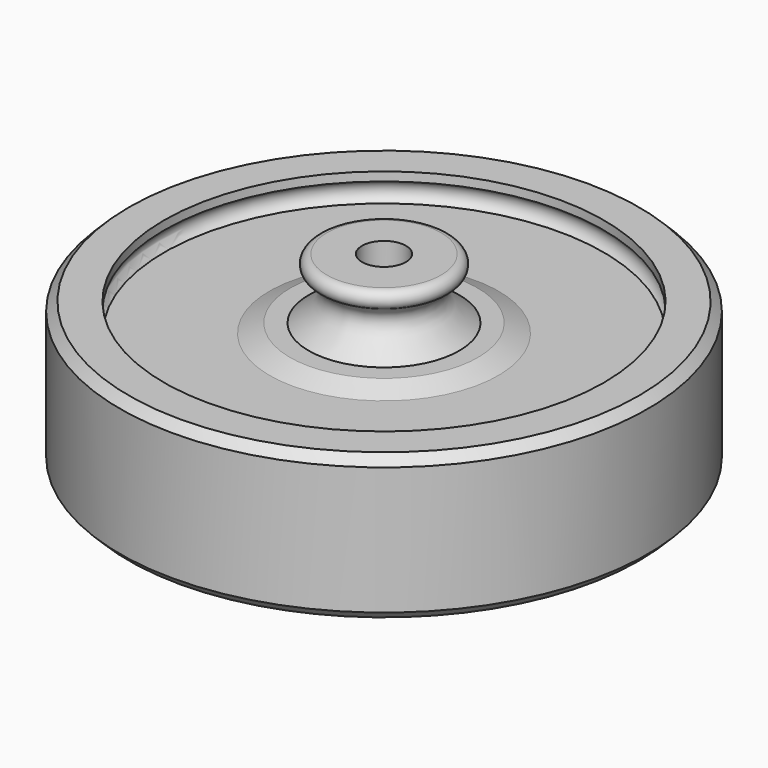
from build123d import *

# Parameters (mm, degrees)
F2_SIZE  = 1
F4_D     = 5
F4_DEPTH = 8
F4_TIP   = 1.5021515476
F6_D     = 5
F6_DEPTH = 8
F6_TIP   = 1.5021515476


# Not quite as in the source:
# - a feature names something its author has since deleted; it is built from what else it names


with BuildPart() as f1:
    # F0 (on Right) → F1 (revolve)
    with BuildSketch(Plane.YZ):
        with BuildLine():
            Line((0, 13.0073325709), (-6.4953151159, 13.0073325709))
            ThreePointArc((-6.4953151159, 13.0073325709), (-7.4722561915, 12.0045412332), (-6.4953151159, 11.0017498955))
            add(Edge.make_bspline(
                [(-6.4953151159, 11.0017498955), (-6.1929281207, 10.6202125837), (-5.580196849, 9.8470978466), (-5.8469313962, 8.0940443784), (-7.5430271882, 6.8547624607), (-8.5644554347, 6.1084381305)],
                knots=[0, 0, 0, 0, 0.2793196515, 0.5659895696, 1, 1, 1, 1], degree=3))
            Line((-8.5644554347, 6.1084381305), (-10.6689063832, 6.1084381305))
            Line((-10.6689063832, 6.1084381305), (-13.0015872419, 5.0749718212))
            Line((-13.0015872419, 5.0749718212), (-24.9405857176, 5.0749718212))
            ThreePointArc((-24.9405857176, 5.0749718212), (-25.5901300386, 6.1484332461), (-24.989798665, 7.2501725517))
            Line((-24.989798665, 7.2501725517), (-24.989798665, 8.2541117445))
            Line((-24.989798665, 8.2541117445), (-29.9844965339, 8.2541117445))
            Line((-29.9844965339, 8.2541117445), (-29.9844965339, -8.2651954144))
            Line((-29.9844965339, -8.2651954144), (-24.9865408987, -8.2651954144))
            Line((-24.9865408987, -8.2651954144), (-24.9865408987, -7.2585809976))
            ThreePointArc((-24.9865408987, -7.2585809976), (-25.5762810193, -6.1635660678), (-24.9631311744, -5.0814854912))
            Line((-24.9631311744, -5.0814854912), (-12.9891019315, -5.0814854912))
            Line((-12.9891019315, -5.0814854912), (-10.6949573383, -6.1115091667))
            Line((-10.6949573383, -6.1115091667), (-8.5644554347, -6.1115091667))
            add(Edge.make_bspline(
                [(-8.5644554347, -6.1115091667), (-7.5391964524, -6.9501185029), (-6.0044956131, -8.2054251856), (-5.595225451, -9.0898659277), (-5.7068148514, -9.8706956249), (-6.1934289739, -10.5853317949), (-6.478224881, -11.0035799444)],
                knots=[0, 0, 0, 0, 0.3859396697, 0.577709579, 0.7528501991, 1, 1, 1, 1], degree=3))
            ThreePointArc((-6.478224881, -11.0035799444), (-7.4583694346, -12.0006089311), (-6.4953151159, -13.01415544))
            Line((-6.4953151159, -13.01415544), (0, -13.01415544))
            Line((0, -13.01415544), (0, 13.0073325709))
        make_face()
    revolve(axis=Axis((0, 0, -0.0034114346), (0, 0, -1)))

    # F2
    f2_edges = [f1.edges().sort_by_distance(p)[0] for p in [
        (0, 29.984497, 8.254112),
        (0, 29.984497, -8.265195),
    ]]
    chamfer(f2_edges, length=F2_SIZE)

    # F4
    with Locations(Plane.XY.offset(13.0073325709)):
        with Locations((0, 0)):
            Hole(F4_D / 2, depth=F4_DEPTH)
            with Locations((0, 0, -(F4_DEPTH + F4_TIP / 2))):  # 118° drill point
                Cone(0, F4_D / 2, F4_TIP, mode=Mode.SUBTRACT)

    # F6
    with Locations(Plane(origin=(0, 0, -13.01415544), x_dir=(1, 0, 0), z_dir=(0, 0, -1))):
        with Locations((0, 0)):
            Hole(F6_D / 2, depth=F6_DEPTH)
            with Locations((0, 0, -(F6_DEPTH + F6_TIP / 2))):  # 118° drill point
                Cone(0, F6_D / 2, F6_TIP, mode=Mode.SUBTRACT)


solid = f1.part
